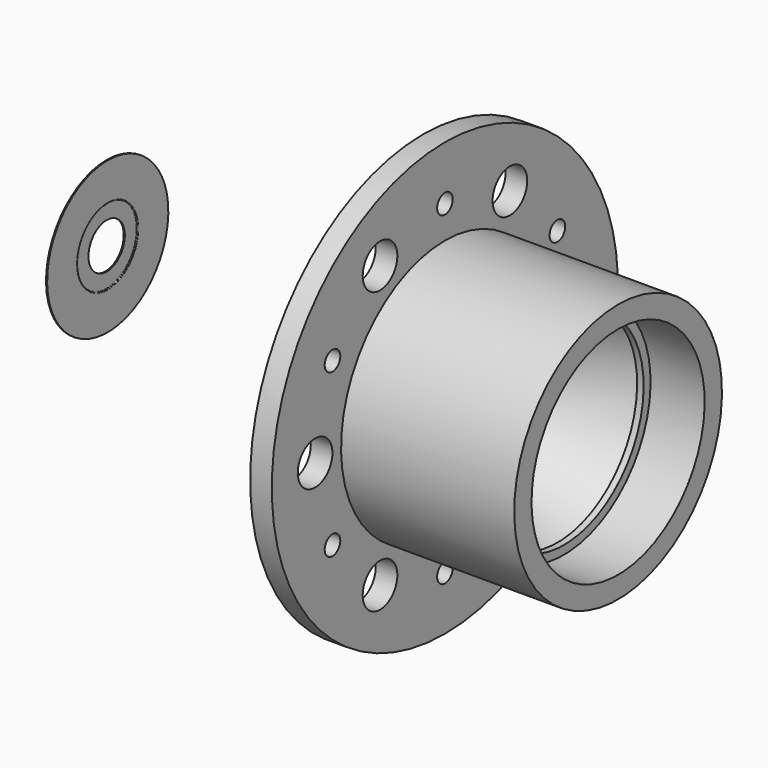
from build123d import *

# Parameters (mm, degrees)
F3_D            = 9
F3_COPIES_COUNT = 6
F4_D            = 20
F4_COPIES_COUNT = 6


# Not quite as in the source:
# - a pattern or mirror of a feature is missing from the dataset's text; its kind, count and spacing are read off the source's solid


with BuildPart() as f1:
    # F0 (on Front) → F1 (revolve)
    with BuildSketch(Plane.XZ):
        Polygon((0, 38), (0, 36), (19, 36), (19, 32), (22, 32), (22, 36), (62, 50), (62, 46), (65, 46), (65, 50), (90, 50), (90, 60), (10, 60), (10, 100), (0, 100), (0, 43), (-4, 43), (-4, 38), align=None)
    revolve(axis=Axis((0.1010708511, 0, 0), (1, 0, 0)))

    # F3 (through all)
    with Locations(Plane(origin=(0, 0, 0), x_dir=(0, -1, 0), z_dir=(-1, 0, 0))):
        with Locations((0, 75)):
            f3 = Hole(F3_D / 2)

    # F3_copies: F3 ×6 about axis
    f3_copies_axis = Axis((0, 0, 0), (1, 0, 0))
    for i in range(1, F3_COPIES_COUNT):
        add(f3.rotate(f3_copies_axis, i * 360 / F3_COPIES_COUNT), mode=Mode.SUBTRACT)

    # F4 (through all)
    with Locations(Plane(origin=(0, 0, 0), x_dir=(0, -1, 0), z_dir=(-1, 0, 0))):
        with Locations((-37.5, 64.9519052838)):
            f4 = Hole(F4_D / 2)

    # F4_copies: F4 ×6 about axis
    f4_copies_axis = Axis((0, 0, 0), (1, 0, 0))
    for i in range(1, F4_COPIES_COUNT):
        add(f4.rotate(f4_copies_axis, i * 360 / F4_COPIES_COUNT), mode=Mode.SUBTRACT)


with BuildPart() as f6:
    # F5 (on Front) → F6 (revolve)
    with BuildSketch(Plane.XZ):
        with BuildLine():
            Line((-146.8164175749, 24.7147989739), (-146.8164175749, 17.4647989739))
            Line((-146.8164175749, 17.4647989739), (-146.3164175749, 17.4647989739))
            Line((-146.3164175749, 17.4647989739), (-146.3164175749, 24.2147989739))
            ThreePointArc((-146.3164175749, 24.2147989739), (-146.2431942702, 24.3915756692), (-146.0664175749, 24.4647989739))
            ThreePointArc((-146.0664175749, 24.4647989739), (-145.8896408796, 24.5380222786), (-145.8164175749, 24.7147989739))
            Line((-145.8164175749, 24.7147989739), (-145.8164175749, 41.9647989739))
            Line((-145.8164175749, 41.9647989739), (-146.3164175749, 41.9647989739))
            Line((-146.3164175749, 41.9647989739), (-146.3164175749, 25.2147989739))
            ThreePointArc((-146.3164175749, 25.2147989739), (-146.3896408796, 25.0380222786), (-146.5664175749, 24.9647989739))
            ThreePointArc((-146.5664175749, 24.9647989739), (-146.7431942702, 24.8915756692), (-146.8164175749, 24.7147989739))
        make_face()
    revolve(axis=Axis((-146.5664175749, 0, 6.9647989739), (1, 0, 0)))


solid = Compound([f1.part, f6.part])
